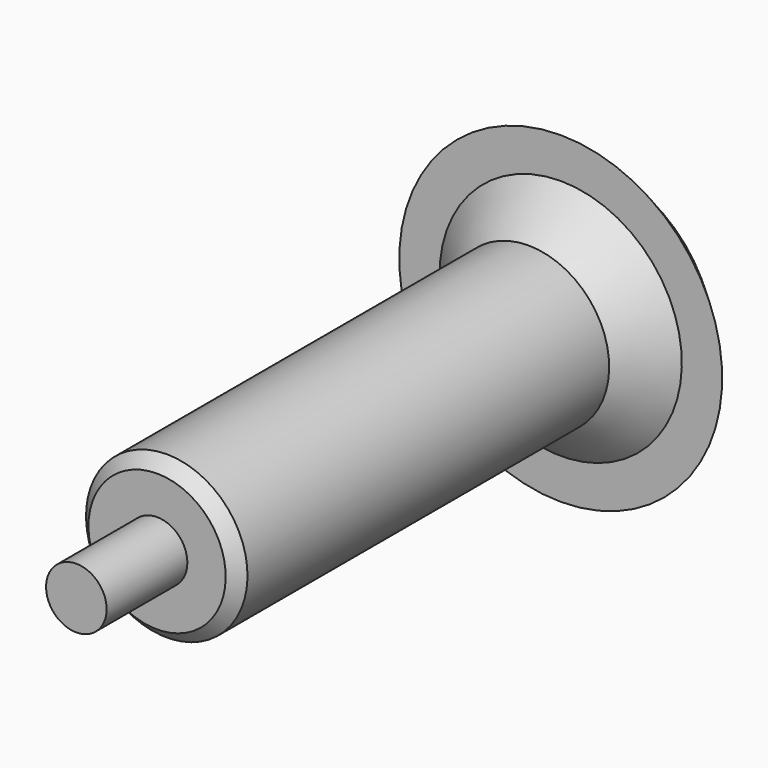
from build123d import *

# Parameters (mm, degrees)
F2_SIZE = 3
F3_SIZE = 10
F4_SIZE = 9.99999


# Not quite as in the source:
# - a fillet or chamfer is up to 0.001 mm smaller than in the source, because OpenCascade refuses the exact size


with BuildPart() as f1:
    # F0 (on Right) → F1 (revolve)
    with BuildSketch(Plane.YZ):
        Polygon((-160, 0), (0, 0), (0, 40), (-10, 40), (-10, 20), (-135, 20), (-135, 7.5), (-160, 7.5), align=None)
    revolve(axis=Axis((0, -33.7878718802, 0), (0, 1, 0)))

    # F2
    f2_edges = [f1.edges().sort_by_distance(p)[0] for p in [
        (0, -135, -20),
    ]]
    chamfer(f2_edges, length=F2_SIZE)

    # F3
    f3_edges = [f1.edges().sort_by_distance(p)[0] for p in [
        (0, -10, -20),
    ]]
    chamfer(f3_edges, length=F3_SIZE)

    # F4 (size 10 in the source; OpenCascade refuses exactly that, so slightly less here)
    f4_edges = [f1.edges().sort_by_distance(p)[0] for p in [
        (0, 0, -40),
    ]]
    chamfer(f4_edges, length=F4_SIZE)


solid = f1.part
